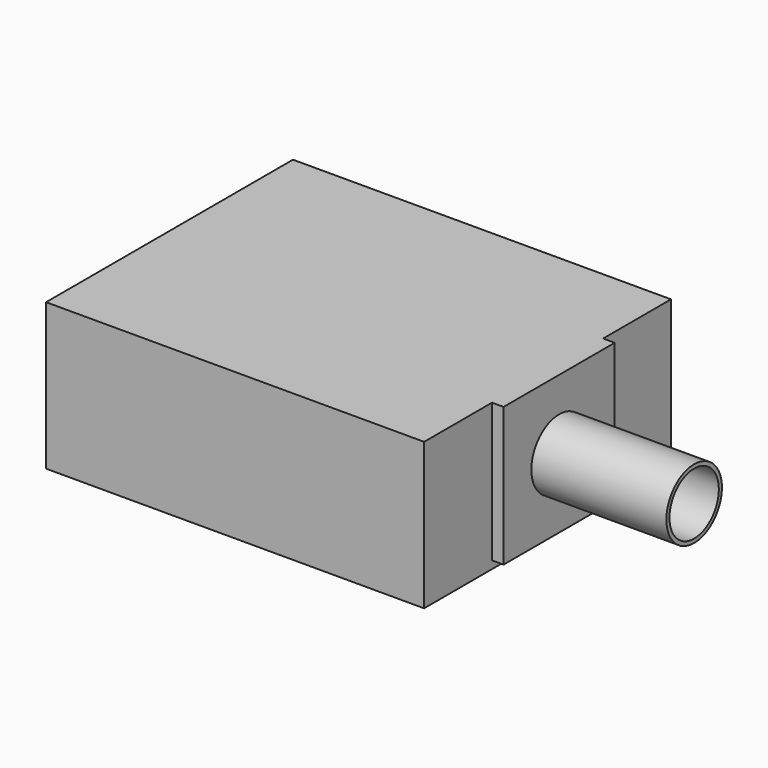
from build123d import *

# Parameters (mm, degrees)
F0_W        = 49
F0_H        = 19
F1_DEPTH    = 20
F2_R        = 4.5
F3_DEPTH    = 1.5
F4_DEPTH    = 19
F5_T        = 0.5
F5_T3_DEPTH = 19
F5_T5_DEPTH = 19


# Not quite as in the source:
# - a shell that OpenCascade refuses in one call is made with other operations: the cavity is built on its own and cut out


with BuildPart() as f1:
    # F0 (on Front) → F1 (new body, symmetric)
    with BuildSketch(Plane.XZ):
        with Locations((1.5, 9.5)):
            Rectangle(F0_W, F0_H)
    extrude(amount=F1_DEPTH, both=True)

    # F2 (on face) → F3 (join)
    with BuildSketch(Plane.YZ.offset(26)):
        Polygon((-9, 19), (-9, 1), (0, 1), (9, 1), (9, 19), (0, 19), align=None)
        with Locations((0, 10)):
            Circle(F2_R, mode=Mode.SUBTRACT)
    extrude(amount=F3_DEPTH)

    # F4 (add): a face of the model
    f4_faces = [f1.faces().sort_by_distance(p)[0] for p in [
        (26, 0, 10),
    ]]
    extrude(f4_faces, amount=F4_DEPTH)

    # F5: shell of thickness 0.5, made by hand


with BuildPart() as f5_core1:
    # F5_t2: copy of F1
    add(f1.part)

    # the walls: a layer under each face that stays
    f5_faces = [f5_core1.faces().sort_by_distance(p)[0] for p in [
        (2.25, 0, 19),
        (1.5, 20, 9.5),
        (-23, 0, 9.5),
        (1.5, -20, 9.5),
        (26, 13.3333333333, 3.1666666667),
        (26.75, -9, 10),
        (27.5, -6, 4),
        (26.75, 9, 10),
        (1.5, 0, 0),
        (26.75, 0, 1),
        (36.25, -4.5, 10),
    ]]
    thicken(f5_faces, amount=-F5_T, mode=Mode.SUBTRACT)

    # F5_s4 → F5_t3 (cut)
    with BuildSketch(Plane.XY.offset(0.5)):
        Polygon((26.005, -9.005), (25.5, -9), (25.5, -8.5), (26, -8.5), align=None)
        Polygon((26.005, 9.005), (25.5, 9), (25.5, 8.5), (26, 8.5), align=None)
    extrude(amount=F5_T3_DEPTH, mode=Mode.SUBTRACT)

    # F5_s6 → F5_t5 (cut)
    with BuildSketch(Plane.XZ.offset(-9.5)):
        Polygon((26.005, 0.995), (25.5, 1), (25.5, 1.5), (26, 1.5), align=None)
    extrude(amount=F5_T5_DEPTH, mode=Mode.SUBTRACT)

    # F5_s7 → F5_t8 (revolve, cut)
    with BuildSketch(Plane.XY.offset(10)):
        Polygon((27.505, 4.505), (27, 4.5), (27, 4), (27.5, 4), align=None)
    revolve(axis=Axis((27.5, 0, 10), (1, 0, 0)), mode=Mode.SUBTRACT)


with BuildPart() as f1_1:
    add(f1.part)

    # what is left inside the walls is the cavity
    f5_cavity = [f5_core1.part.solids().sort_by_distance(p)[0] for p in [
        (2.25, 6.5, 18.495),
    ]]
    add(f5_cavity, mode=Mode.SUBTRACT)


solid = f1_1.part
